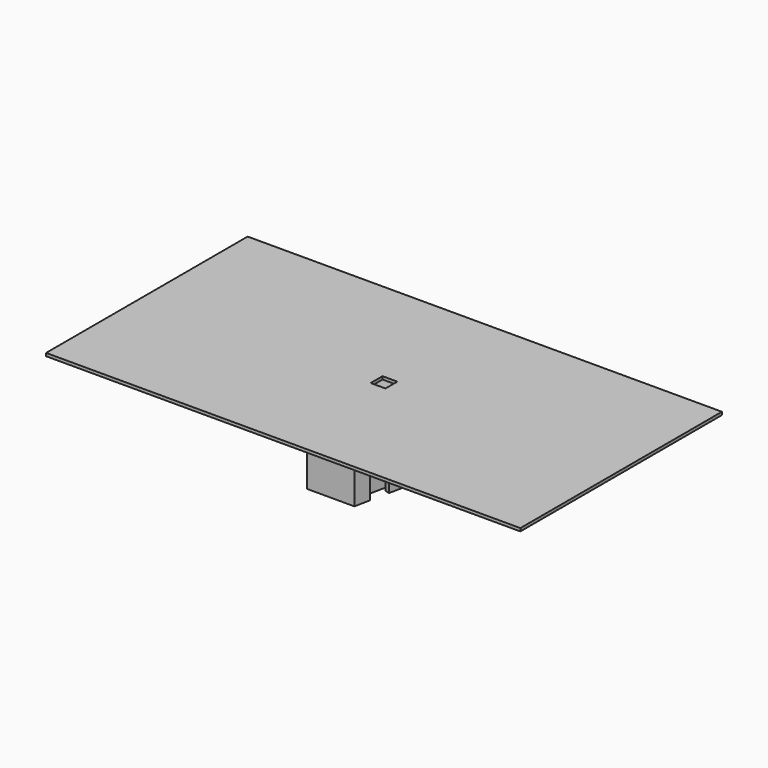
from build123d import *

# Parameters (mm, degrees)
F0_W      = 160
F0_H      = 85
F0_R      = 8
F1_DEPTH  = 1
F3_R      = 8
F4_DEPTH  = 24.1
F6_DEPTH  = 8.7145
F8_DEPTH  = 8.175
F10_DEPTH = 8.715
F12_DEPTH = 8.715
F13_W     = 5
F13_H     = 5
F14_DEPTH = 25
F16_DEPTH = 34.8
F17_R     = 1
F19_R     = 1.5
F20_DEPTH = 8.88


# Not quite as in the source:
# - a feature of the source that left no trace in its solid (it failed there, or was rolled back) is left out


with BuildPart() as f1:
    # F0 (on Top) → F1 (new body)
    with BuildSketch(Plane.XY):
        Rectangle(F0_W, F0_H)
        Circle(F0_R, mode=Mode.SUBTRACT)
        Circle(F0_R)
    extrude(amount=F1_DEPTH)

    # F3 (on face) → F4 (join)
    with BuildSketch(Plane(origin=(0, 0, 0), x_dir=(1, 0, 0), z_dir=(0, 0, -1))):
        Polygon((10.7943351377, -8.8776162038), (12, -3), (12, 3), (11.1962234251, 6.9184108026), (10.3924468502, 10.8368216051), (8.9230427993, 10.5354053895), (9.3249310867, 8.5761999883), (7.8555270357, 8.2747837727), (5.7456135267, 18.5606121294), (7.2150175776, 18.862028345), (7.6169058651, 16.9028229437), (9.086309916, 17.2042391593), (8, 22.5), (-8, 22.5), (-9.086309916, 17.2042391593), (-7.6169058651, 16.9028229437), (-7.2150175776, 18.862028345), (-5.7456135267, 18.5606121294), (-7.8555270357, 8.2747837727), (-9.3249310867, 8.5761999883), (-8.9230427993, 10.5354053895), (-10.3924468502, 10.8368216051), (-11.1962234251, 6.9184108026), (-12, 3), (-12, -3), (-11.1962234251, -6.9184108026), (-10.3924468502, -10.8368216051), (-8.9230427993, -10.5354053895), (-9.3249310867, -8.5761999883), (-7.8555270357, -8.2747837727), (-5.7456135267, -18.5606121294), (-7.2150175776, -18.862028345), (-7.6169058651, -16.9028229437), (-9.086309916, -17.2042391593), (-8, -22.5), (8, -22.5), (8.9858378442, -17.6940405096), (9.086309916, -17.2042391593), (7.6169058651, -16.9028229437), (7.2150175776, -18.862028345), (5.7456135267, -18.5606121294), (7.8555270357, -8.2747837727), (9.3249310867, -8.5761999883), (8.9230427993, -10.5354053895), (10.3924468502, -10.8368216051), align=None)
        Circle(F3_R, mode=Mode.SUBTRACT)
    extrude(amount=F4_DEPTH)

    # F5 (on face) → F6 (cut)
    with BuildSketch(Plane(origin=(9.1671855889, 1.8804483259, 0), x_dir=(-0.2009441437, 0.9796027006, 0), z_dir=(0.9796027006, 0.2009441437, 0))):
        with BuildLine():
            ThreePointArc((13.2774783773, -11.45), (12.838138549, -10.3893398282), (11.7774783773, -9.95))
            ThreePointArc((11.7774783773, -9.95), (10.7168182055, -12.5106601718), (13.2774783773, -11.45))
        make_face()
    extrude(amount=-F6_DEPTH, mode=Mode.SUBTRACT)

    # F7 (on face) → F8 (cut)
    with BuildSketch(Plane(origin=(-9.1671855889, 1.8804483259, 0), x_dir=(-0.2009441437, -0.9796027006, 0), z_dir=(-0.9796027006, 0.2009441437, 0))):
        with BuildLine():
            ThreePointArc((-10.2774783773, -11.45), (-10.7168182055, -10.3893398282), (-11.7774783773, -9.95))
            ThreePointArc((-11.7774783773, -9.95), (-12.838138549, -12.5106601718), (-10.2774783773, -11.45))
        make_face()
    extrude(amount=-F8_DEPTH, mode=Mode.SUBTRACT)

    # F9 (on face) → F10 (cut)
    with BuildSketch(Plane(origin=(-9.1671855889, -1.8804483259, 0), x_dir=(0.2009441437, -0.9796027006, 0), z_dir=(-0.9796027006, -0.2009441437, 0))):
        with BuildLine():
            ThreePointArc((11.7774783773, -9.95), (10.7168182055, -12.5106601718), (13.2774783773, -11.45))
            ThreePointArc((13.2774783773, -11.45), (12.838138549, -10.3893398282), (11.7774783773, -9.95))
        make_face()
    extrude(amount=-F10_DEPTH, mode=Mode.SUBTRACT)

    # F11 (on face) → F12 (cut)
    with BuildSketch(Plane(origin=(9.1671855889, -1.8804483259, 0), x_dir=(0.2009441437, 0.9796027006, 0), z_dir=(0.9796027006, -0.2009441437, 0))):
        with BuildLine():
            ThreePointArc((-11.7774783773, -9.95), (-12.838138549, -12.5106601718), (-10.2774783773, -11.45))
            ThreePointArc((-10.2774783773, -11.45), (-10.7168182055, -10.3893398282), (-11.7774783773, -9.95))
        make_face()
    extrude(amount=-F12_DEPTH, mode=Mode.SUBTRACT)

    # F13 (on face) → F14 (cut)
    with BuildSketch(Plane(origin=(0, 0, 0), x_dir=(1, 0, 0), z_dir=(0, 0, -1))):
        Rectangle(F13_W, F13_H)
    extrude(amount=-F14_DEPTH, mode=Mode.SUBTRACT)

    # F15 (on face) → F16 (cut)
    with BuildSketch(Plane.XZ.offset(22.5)):
        with BuildLine():
            ThreePointArc((0, -10.55), (-1.5, -12.05), (0, -13.55))
            Line((0, -13.55), (0, -12.05))
            Line((0, -12.05), (0, -10.55))
        make_face()
        with BuildLine():
            Line((0, -12.05), (0, -13.55))
            ThreePointArc((0, -13.55), (1.0606601718, -13.1106601718), (1.5, -12.05))
            ThreePointArc((1.5, -12.05), (1.0606601718, -10.9893398282), (0, -10.55))
            Line((0, -10.55), (0, -12.05))
        make_face()
    extrude(amount=-F16_DEPTH, mode=Mode.SUBTRACT)

    # F17
    f17_edges = [f1.edges().sort_by_distance(p)[0] for p in [
        (8, 0, -12.05),
        (0, -8, -10.55),
        (0, 8, -10.55),
    ]]
    fillet(f17_edges, radius=F17_R)

    # F19 (on face) → F20 (join)
    with BuildSketch(Plane.XZ.offset(22.5)):
        with Locations((0, -12.05)):
            Circle(F19_R)
    extrude(amount=-F20_DEPTH)


solid = f1.part
